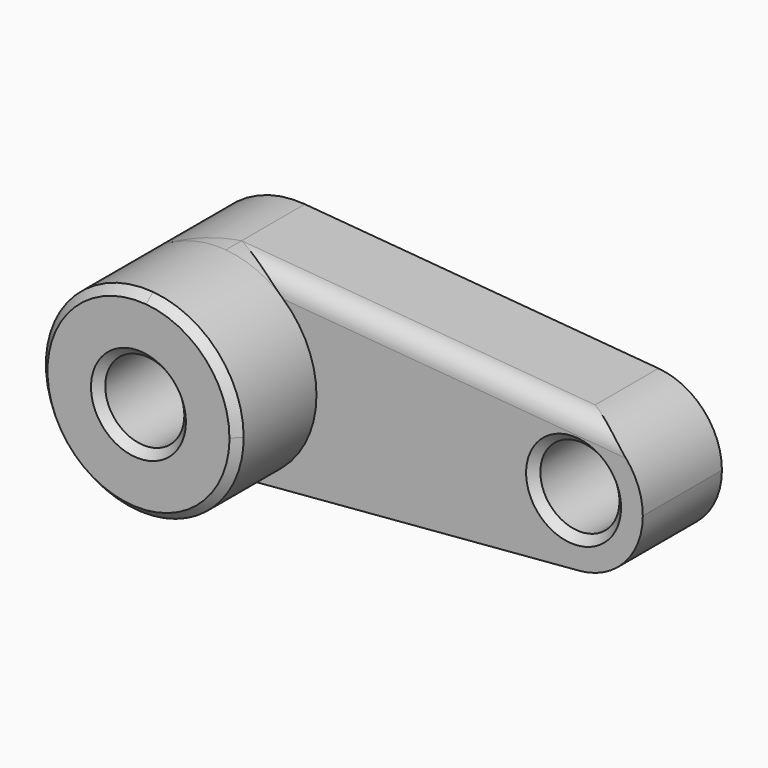
from build123d import *

# Parameters (mm, degrees)
F0_R        = 10
F1_DEPTH    = 25
F2_DEPTH    = 50
F3_SIZE     = 2
F4_T4_DEPTH = 123.4369555733
F4_S5_R     = 25
F4_T6_DEPTH = 64


# Not quite as in the source:
# - a fillet or chamfer that OpenCascade refuses, or shapes differently, is made with other operations: its cross-section is extruded or revolved along the edge and cut away or added


with BuildPart() as f1:
    # F0 (on Front) → F1 (new body)
    with BuildSketch(Plane.XZ):
        with BuildLine():
            ThreePointArc((2.0833333333, -24.9130432148), (18.3995018048, -16.9250800097), (25, 0))
            ThreePointArc((25, 0), (18.3995018048, 16.9250800097), (2.0833333333, 24.9130432148))
            ThreePointArc((2.0833333333, 24.9130432148), (-25, 0), (2.0833333333, -24.9130432148))
        make_face()
        Circle(F0_R, mode=Mode.SUBTRACT)
        with BuildLine():
            ThreePointArc((2.0833333333, 24.9130432148), (18.3995018048, 16.9250800097), (25, 0))
            ThreePointArc((25, 0), (18.3995018048, -16.9250800097), (2.0833333333, -24.9130432148))
            Line((2.0833333333, -24.9130432148), (91.4583333333, -17.4391302504))
            ThreePointArc((91.4583333333, -17.4391302504), (72.5, 0), (91.4583333333, 17.4391302504))
            Line((91.4583333333, 17.4391302504), (2.0833333333, 24.9130432148))
        make_face()
        with BuildLine():
            ThreePointArc((107.5, 0), (102.8796512634, 11.8475560068), (91.4583333333, 17.4391302504))
            ThreePointArc((91.4583333333, 17.4391302504), (72.5, 0), (91.4583333333, -17.4391302504))
            ThreePointArc((91.4583333333, -17.4391302504), (102.8796512634, -11.8475560068), (107.5, 0))
        make_face()
        with Locations((90, 0)):
            Circle(F0_R, mode=Mode.SUBTRACT)
    extrude(amount=F1_DEPTH)

    # F0 (on Front) → F2 (join)
    with BuildSketch(Plane.XZ):
        with BuildLine():
            ThreePointArc((2.0833333333, -24.9130432148), (18.3995018048, -16.9250800097), (25, 0))
            ThreePointArc((25, 0), (18.3995018048, 16.9250800097), (2.0833333333, 24.9130432148))
            ThreePointArc((2.0833333333, 24.9130432148), (-25, 0), (2.0833333333, -24.9130432148))
        make_face()
        Circle(F0_R, mode=Mode.SUBTRACT)
    extrude(amount=F2_DEPTH)

    # F3
    f3_edges = [f1.edges().sort_by_distance(p)[0] for p in [
        (-2.083333, -50, 24.913043),
        (-10, -50, 0),
        (80, -25, 0),
    ]]
    chamfer(f3_edges, length=F3_SIZE)

    # F4: fillet of radius 5 on 1 edges, made by hand


with BuildPart() as f4_tool2:
    # F4_s3 → F4_t4 (new body)
    with BuildSketch(Plane(origin=(101.8315216074, 0, -8.5155796311), x_dir=(0, 1, 0), z_dir=(-0.9965217286, 0, 0.0833333333))):
        with BuildLine():
            ThreePointArc((-25, -20), (-23.5355339059, -23.5355339059), (-20, -25))
            Line((-20, -25), (-25, -25))
            Line((-25, -25), (-25, -20))
        make_face()
    extrude(amount=F4_T4_DEPTH)

    # F4_s5 → F4_t6 (cut, symmetric)
    with BuildSketch(Plane.XZ.offset(22.5)):
        Circle(F4_S5_R)
    extrude(amount=F4_T6_DEPTH, both=True, mode=Mode.SUBTRACT)


with BuildPart() as f1_1:
    add(f1.part)

    # F4_t1: cut F4_tool2
    add(f4_tool2.part, mode=Mode.SUBTRACT)


solid = f1_1.part
